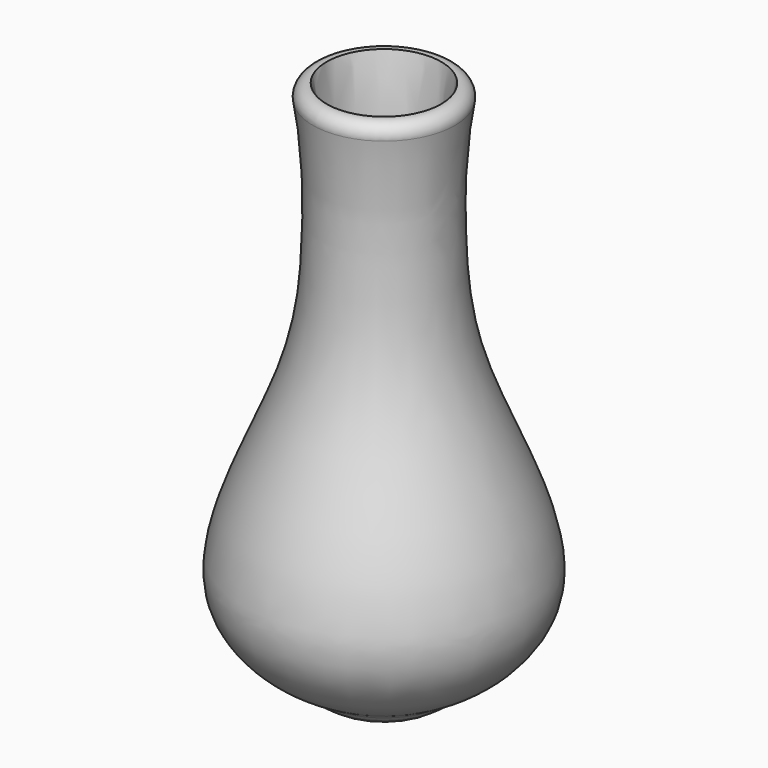
from build123d import *

# Parameters (mm, degrees)
F2_T = -2.54


# Not quite as in the source:
# - a fillet or chamfer that OpenCascade refuses, or shapes differently, is made with other operations: its cross-section is extruded or revolved along the edge and cut away or added


with BuildPart() as f1:
    # F0 (on Front) → F1 (revolve)
    with BuildSketch(Plane.XZ):
        with BuildLine():
            Line((0, 82.8496217728), (0, 0))
            add(Edge.make_bspline(
                [(0, 0), (3.5304676591, 0.5580132439), (7.1007808259, 1.0956639344), (11.0122608021, 2.9600756243)],
                knots=[0, 0, 0, 0, 0.1540172593, 0.1540172593, 0.1540172593, 0.1540172593], degree=3))
            add(Edge.make_bspline(
                [(11.0122608021, 2.9600756243), (11.2513979375, 3.0740606309), (11.4918102738, 3.1930047563), (11.7328625432, 3.3168929744)],
                knots=[0.1540172593, 0.1540172593, 0.1540172593, 0.1540172593, 0.1634334513, 0.1634334513, 0.1634334513, 0.1634334513], degree=3))
            add(Edge.make_bspline(
                [(11.7328625432, 3.3168929744), (16.2066561112, 5.6161881222), (27.5345413493, 15.2743635428), (11.1159696099, 43.5598033465), (9.665282517, 62.9147427418), (9.9363927022, 77.2008571625), (11.6142209154, 84.323503077)],
                knots=[0.1634334513, 0.1634334513, 0.1634334513, 0.1634334513, 0.3381926396, 0.5851546258, 0.7907268611, 1, 1, 1, 1], degree=3))
            ThreePointArc((11.6142209154, 84.323503077), (5.8434931929, 83.2998655771), (0, 82.8496217728))
        make_face()
        with BuildLine():
            add(Edge.make_bspline(
                [(0, 0), (3.5304676591, 0.5580132439), (7.1007808259, 1.0956639344), (11.0122608021, 2.9600756243)],
                knots=[0, 0, 0, 0, 0.1540172593, 0.1540172593, 0.1540172593, 0.1540172593], degree=3))
            Line((0, 0), (5.287025824, 0))
            ThreePointArc((5.287025824, 0), (7.5357843244, 0.4115165903), (9.4930778073, 1.5927290687))
            add(Edge.make_bspline(
                [(9.4930778073, 1.5927290687), (9.7925324175, 1.8574862531), (10.0914061082, 2.1222705155), (10.3856044775, 2.3872727055)],
                knots=[2.3827711581, 2.3827711581, 2.3827711581, 2.3827711581, 3.5719284125, 3.5719284125, 3.5719284125, 3.5719284125], degree=3))
            add(Edge.make_bspline(
                [(10.3856044775, 2.3872727055), (10.5974228817, 2.5780702995), (10.8068177005, 2.7689808625), (11.0122608021, 2.9600756243)],
                knots=[3.5719284125, 3.5719284125, 3.5719284125, 3.5719284125, 4.4281037635, 4.4281037635, 4.4281037635, 4.4281037635], degree=3))
        make_face()
        with BuildLine():
            add(Edge.make_bspline(
                [(11.0122608021, 2.9600756243), (11.2513979375, 3.0740606309), (11.4918102738, 3.1930047563), (11.7328625432, 3.3168929744)],
                knots=[0.1540172593, 0.1540172593, 0.1540172593, 0.1540172593, 0.1634334513, 0.1634334513, 0.1634334513, 0.1634334513], degree=3))
            add(Edge.make_bspline(
                [(10.3856044775, 2.3872727055), (10.5974228817, 2.5780702995), (10.8068177005, 2.7689808625), (11.0122608021, 2.9600756243)],
                knots=[3.5719284125, 3.5719284125, 3.5719284125, 3.5719284125, 4.4281037635, 4.4281037635, 4.4281037635, 4.4281037635], degree=3))
            ThreePointArc((10.3856044775, 2.3872727055), (11.0291542381, 2.8956754158), (11.7328625432, 3.3168929744))
        make_face()
    revolve(axis=Axis((0, 0, 43.3439351618), (0, 0, 1)))

    # F2
    f2_openings = [f1.faces().sort_by_distance(p)[0] for p in [
        (-5.843493, 0, 83.299866),
    ]]
    offset(amount=F2_T, openings=f2_openings, kind=Kind.INTERSECTION)

    # F3: fillet of radius 1.905 on 1 edges, made by hand

    # F3_s1 → F3_t2 (revolve, cut)
    with BuildSketch(Plane.XZ):
        with BuildLine():
            ThreePointArc((11.0348110205, 81.5402492032), (10.531170729, 83.2042706578), (8.8859569598, 83.7663138931))
            Line((8.8859569598, 83.7663138931), (8.8804646475, 83.8040159422))
            ThreePointArc((8.8804646475, 83.8040159422), (10.2457291095, 84.0662562823), (11.6057247131, 84.3606436821))
            Line((11.6057247131, 84.3606436821), (11.6513058893, 84.3147672482))
            ThreePointArc((11.6513058893, 84.3147672482), (11.3439338902, 82.9278378574), (11.0722957894, 81.5334299585))
            Line((11.0722957894, 81.5334299585), (11.0348110205, 81.5402492032))
        make_face()
    revolve(axis=Axis((0, 0, 84.323503077), (0, 0, 1)), mode=Mode.SUBTRACT)


solid = f1.part
